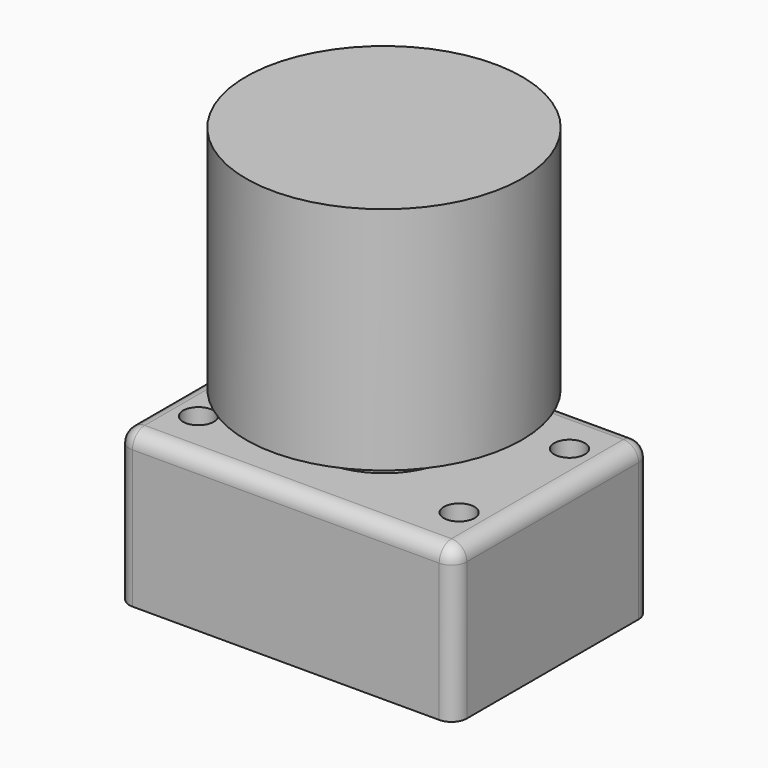
from build123d import *

# Parameters (mm, degrees)
F0_W      = 15
F0_H      = 14
F0_W_2    = 13
F0_H_2    = 12
F1_DEPTH  = 6
F2_W      = 6
F2_H      = 12
F3_DEPTH  = 1.5
F4_W      = 13
F4_H      = 12
F5_DEPTH  = 4.5
F6_R      = 3.5
F7_DEPTH  = 7
F8_R      = 3
F9_DEPTH  = 13.5
F11_DEPTH = 10
F12_W     = 22
F12_H     = 16
F12_W_2   = 20
F12_H_2   = 14
F13_DEPTH = 8
F14_W     = 22
F14_H     = 16
F14_R     = 1
F14_R_2   = 4.5
F15_DEPTH = 2
F16_R     = 1
F18_R     = 5.5
F18_R_2   = 3.5
F19_DEPTH = 2
F20_R     = 4.5
F20_R_2   = 3.5
F21_DEPTH = 18.5
F23_DEPTH = 9
F24_R     = 4.5
F25_DEPTH = 1
F26_R     = 9
F26_R_2   = 3.5
F27_DEPTH = 15


with BuildPart() as f1:
    # F0 (on Top) → F1 (new body)
    with BuildSketch(Plane.XY):
        Rectangle(F0_W, F0_H)
        Rectangle(F0_W_2, F0_H_2, mode=Mode.SUBTRACT)
    extrude(amount=F1_DEPTH)

    # F2 (on Top) → F3 (join)
    with BuildSketch(Plane.XY):
        Rectangle(F2_W, F2_H)
    extrude(amount=F3_DEPTH)


with BuildPart() as f5:
    # F4 (on face) → F5 (new body)
    with BuildSketch(Plane.XY.offset(1.5)):
        Rectangle(F4_W, F4_H)
    extrude(amount=F5_DEPTH)

    # F6 (on face) → F7 (join)
    with BuildSketch(Plane.XY.offset(6)):
        Circle(F6_R)
    extrude(amount=F7_DEPTH)

    # F8 (on face) → F9 (join)
    with BuildSketch(Plane.XY.offset(13)):
        Circle(F8_R)
    extrude(amount=F9_DEPTH)

    # F10 (on face) → F11 (cut)
    with BuildSketch(Plane.XY.offset(26.5)):
        with BuildLine():
            Line((2.5980762114, -1.5), (-2.5980762114, -1.5))
            ThreePointArc((-2.5980762114, -1.5), (0, -3), (2.5980762114, -1.5))
        make_face()
    extrude(amount=-F11_DEPTH, mode=Mode.SUBTRACT)


with BuildPart() as f13:
    # F12 (on Top) → F13 (new body)
    with BuildSketch(Plane.XY):
        Rectangle(F12_W, F12_H)
        Rectangle(F12_W_2, F12_H_2, mode=Mode.SUBTRACT)
    extrude(amount=F13_DEPTH)

    # F14 (on face) → F15 (join)
    with BuildSketch(Plane.XY.offset(8)):
        Rectangle(F14_W, F14_H)
        with Locations((-8.5, -4.5)):
            Circle(F14_R, mode=Mode.SUBTRACT)
        with Locations((8.5, -4.5)):
            Circle(F14_R, mode=Mode.SUBTRACT)
        with Locations((-8.5, 4.5)):
            Circle(F14_R, mode=Mode.SUBTRACT)
        Circle(F14_R_2, mode=Mode.SUBTRACT)
        with Locations((8.5, 4.5)):
            Circle(F14_R, mode=Mode.SUBTRACT)
    extrude(amount=F15_DEPTH)

    # F16
    f16_edges = [f13.edges().sort_by_distance(p)[0] for p in [
        (-11, -8, 5),
        (11, -8, 5),
        (11, 8, 5),
        (-11, 8, 5),
        (0, -8, 10),
        (0, 8, 10),
        (-11, 0, 10),
        (11, 0, 10),
    ]]
    fillet(f16_edges, radius=F16_R)


with BuildPart() as f19:
    # F18 (on offset) → F19 (new body)
    with BuildSketch(Plane.XY.offset(6)):
        Circle(F18_R)
        Circle(F18_R_2, mode=Mode.SUBTRACT)
    extrude(amount=F19_DEPTH)

    # F20 (on face) → F21 (join)
    with BuildSketch(Plane.XY.offset(8)):
        Circle(F20_R)
        Circle(F20_R_2, mode=Mode.SUBTRACT)
    extrude(amount=F21_DEPTH)

    # F22 (on face) → F23 (join)
    with BuildSketch(Plane.XY.offset(26.5)):
        with BuildLine():
            Line((3.1622776602, -1.5), (-3.1622776602, -1.5))
            ThreePointArc((-3.1622776602, -1.5), (0, -3.5), (3.1622776602, -1.5))
        make_face()
    extrude(amount=-F23_DEPTH)

    # F24 (on face) → F25 (join)
    with BuildSketch(Plane.XY.offset(26.5)):
        Circle(F24_R)
    extrude(amount=F25_DEPTH)

    # F26 (on face) → F27 (join)
    with BuildSketch(Plane.XY.offset(27.5)):
        Circle(F26_R)
        Circle(F26_R_2, mode=Mode.SUBTRACT)
    extrude(amount=-F27_DEPTH)


solid = Compound([f1.part, f5.part, f13.part, f19.part])
